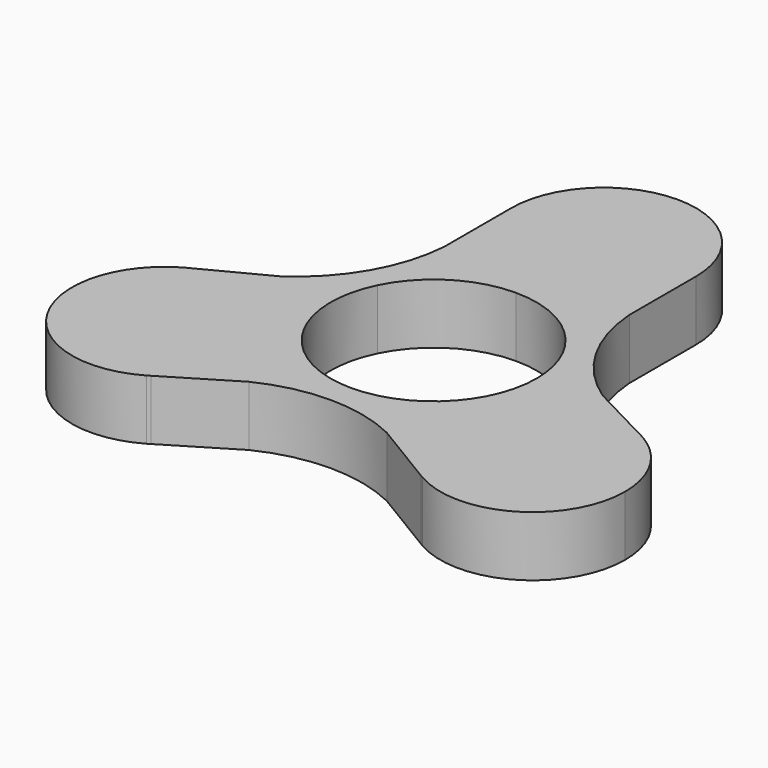
from build123d import *

# Parameters (mm, degrees)
F1_DEPTH = 6.5


# Not quite as in the source:
# - a feature names something its author has since deleted; it is built from what else it names


with BuildPart() as f1:
    # F0 (on Top) → F1 (new body)
    with BuildSketch(Plane.XY):
        with BuildLine():
            Line((10, 13.9658923334), (10, 5.6794919243))
            Line((10, 5.6794919243), (10.6173677664, 4.610179586))
            Line((10.6173677664, 4.610179586), (17.4592921435, 1.0460193523))
            ThreePointArc((17.4592921435, 1.0460193523), (12.2366972109, 6.6440014162), (10, 13.9658923334))
        make_face()
        with BuildLine():
            Line((5, 14.3397459622), (10, 5.6794919243))
            Line((10, 5.6794919243), (10, 13.9658923334))
            Line((10, 13.9658923334), (10, 23))
            ThreePointArc((10, 23), (8.6602540378, 18), (5, 14.3397459622))
        make_face()
        with BuildLine():
            Line((17.4592921435, 1.0460193523), (10.6173677664, 4.610179586))
            Line((10.6173677664, 4.610179586), (14.918584287, -2.8397459622))
            ThreePointArc((14.918584287, -2.8397459622), (19.4852389907, -1.5093938195), (24.1499344795, -2.4393336035))
            Line((24.1499344795, -2.4393336035), (17.4592921435, 1.0460193523))
        make_face()
        with BuildLine():
            Line((-7.4592921435, -15.6551270189), (-0.5795069127, -11.5))
            Line((-0.5795069127, -11.5), (-9.918584287, -11.5))
            ThreePointArc((-9.918584287, -11.5), (-11.1613785992, -16.328182737), (-14.5808539954, -19.9562778652))
            Line((-14.5808539954, -19.9562778652), (-7.4592921435, -15.6551270189))
        make_face()
        with BuildLine():
            Line((0.5795069127, -11.5), (-0.5795069127, -11.5))
            Line((-0.5795069127, -11.5), (-7.4592921435, -15.6551270189))
            ThreePointArc((-7.4592921435, -15.6551270189), (0, -13.9312181655), (7.4592921435, -15.6551270189))
            Line((7.4592921435, -15.6551270189), (0.5795069127, -11.5))
        make_face()
        with BuildLine():
            Line((9.918584287, -11.5), (0.5795069127, -11.5))
            Line((0.5795069127, -11.5), (7.4592921435, -15.6551270189))
            Line((7.4592921435, -15.6551270189), (14.5808539954, -19.9562778652))
            ThreePointArc((14.5808539954, -19.9562778652), (11.1613785992, -16.328182737), (9.918584287, -11.5))
        make_face()
        with BuildLine():
            Line((0, 23), (5, 14.3397459622))
            ThreePointArc((5, 14.3397459622), (8.6602540378, 18), (10, 23))
            Line((10, 23), (0, 23))
        make_face()
        with BuildLine():
            ThreePointArc((24.1499344795, -2.4393336035), (19.4852389907, -1.5093938195), (14.918584287, -2.8397459622))
            Line((14.918584287, -2.8397459622), (19.918584287, -11.5))
            Line((19.918584287, -11.5), (24.918584287, -2.8397459622))
            Line((24.918584287, -2.8397459622), (24.1499344795, -2.4393336035))
        make_face()
        with BuildLine():
            Line((-10, 13.9658923334), (-10, 5.6794919243))
            Line((-10, 5.6794919243), (-5, 14.3397459622))
            ThreePointArc((-5, 14.3397459622), (-8.6602540378, 18), (-10, 23))
            Line((-10, 23), (-10, 13.9658923334))
        make_face()
        with BuildLine():
            Line((-10.6173677664, 4.610179586), (-10, 5.6794919243))
            Line((-10, 5.6794919243), (-10, 13.9658923334))
            ThreePointArc((-10, 13.9658923334), (-12.2366972109, 6.6440014162), (-17.4592921435, 1.0460193523))
            Line((-17.4592921435, 1.0460193523), (-10.6173677664, 4.610179586))
        make_face()
        with BuildLine():
            Line((-14.918584287, -2.8397459622), (-10.6173677664, 4.610179586))
            Line((-10.6173677664, 4.610179586), (-17.4592921435, 1.0460193523))
            Line((-17.4592921435, 1.0460193523), (-24.1499344795, -2.4393336035))
            ThreePointArc((-24.1499344795, -2.4393336035), (-19.4852389907, -1.5093938195), (-14.918584287, -2.8397459622))
        make_face()
        with BuildLine():
            ThreePointArc((-14.5808539954, -19.9562778652), (-11.1613785992, -16.328182737), (-9.918584287, -11.5))
            Line((-9.918584287, -11.5), (-19.918584287, -11.5))
            Line((-19.918584287, -11.5), (-14.918584287, -20.1602540378))
            Line((-14.918584287, -20.1602540378), (-14.5808539954, -19.9562778652))
        make_face()
        with BuildLine():
            Line((19.918584287, -11.5), (9.918584287, -11.5))
            ThreePointArc((9.918584287, -11.5), (11.1613785992, -16.328182737), (14.5808539954, -19.9562778652))
            Line((14.5808539954, -19.9562778652), (14.918584287, -20.1602540378))
            Line((14.918584287, -20.1602540378), (19.918584287, -11.5))
        make_face()
        with BuildLine():
            Line((-5, 14.3397459622), (0, 23))
            Line((0, 23), (-10, 23))
            ThreePointArc((-10, 23), (-8.6602540378, 18), (-5, 14.3397459622))
        make_face()
        with BuildLine():
            Line((-10, 23), (0, 23))
            Line((0, 23), (10, 23))
            ThreePointArc((10, 23), (0, 33), (-10, 23))
        make_face()
        with BuildLine():
            Line((24.918584287, -2.8397459622), (19.918584287, -11.5))
            Line((19.918584287, -11.5), (14.918584287, -20.1602540378))
            ThreePointArc((14.918584287, -20.1602540378), (24.918584287, -20.1602540378), (29.918584287, -11.5))
            ThreePointArc((29.918584287, -11.5), (28.5788383249, -6.5), (24.918584287, -2.8397459622))
        make_face()
        with BuildLine():
            ThreePointArc((24.918584287, -2.8397459622), (24.538599342, -2.6312086003), (24.1499344795, -2.4393336035))
            Line((24.1499344795, -2.4393336035), (24.918584287, -2.8397459622))
        make_face()
        with BuildLine():
            Line((-19.918584287, -11.5), (-14.918584287, -2.8397459622))
            ThreePointArc((-14.918584287, -2.8397459622), (-19.4852389907, -1.5093938195), (-24.1499344795, -2.4393336035))
            Line((-24.1499344795, -2.4393336035), (-24.918584287, -2.8397459622))
            Line((-24.918584287, -2.8397459622), (-19.918584287, -11.5))
        make_face()
        with BuildLine():
            Line((-14.918584287, -20.1602540378), (-19.918584287, -11.5))
            Line((-19.918584287, -11.5), (-24.918584287, -2.8397459622))
            ThreePointArc((-24.918584287, -2.8397459622), (-28.5788383249, -16.5), (-14.918584287, -20.1602540378))
        make_face()
        with BuildLine():
            ThreePointArc((-14.918584287, -20.1602540378), (-14.7487130637, -20.0599317482), (-14.5808539954, -19.9562778652))
            Line((-14.5808539954, -19.9562778652), (-14.918584287, -20.1602540378))
        make_face()
        with BuildLine():
            Line((14.918584287, -20.1602540378), (14.5808539954, -19.9562778652))
            ThreePointArc((14.5808539954, -19.9562778652), (14.7487130637, -20.0599317482), (14.918584287, -20.1602540378))
        make_face()
        with BuildLine():
            Line((-24.918584287, -2.8397459622), (-24.1499344795, -2.4393336035))
            ThreePointArc((-24.1499344795, -2.4393336035), (-24.538599342, -2.6312086003), (-24.918584287, -2.8397459622))
        make_face()
        with BuildLine():
            Line((-0.5795069127, -11.5), (0, -11.15))
            ThreePointArc((0, -11.15), (-9.468682565, -5.8878307111), (-10, 4.9317846668))
            Line((-10, 4.9317846668), (-10.6173677664, 4.610179586))
            Line((-10.6173677664, 4.610179586), (-14.918584287, -2.8397459622))
            ThreePointArc((-14.918584287, -2.8397459622), (-11.2583302492, -6.5), (-9.918584287, -11.5))
            Line((-9.918584287, -11.5), (-0.5795069127, -11.5))
        make_face()
        with BuildLine():
            Line((-19.918584287, -11.5), (-9.918584287, -11.5))
            ThreePointArc((-9.918584287, -11.5), (-11.2583302492, -6.5), (-14.918584287, -2.8397459622))
            Line((-14.918584287, -2.8397459622), (-19.918584287, -11.5))
        make_face()
        Polygon((-10.6173677664, 4.610179586), (-10, 4.9317846668), (-10, 5.6794919243), align=None)
        with BuildLine():
            ThreePointArc((-10, 4.9317846668), (-5.8878307111, 9.468682565), (0, 11.15))
            Line((0, 11.15), (0, 13))
            ThreePointArc((0, 13), (-2.588190451, 13.3407417371), (-5, 14.3397459622))
            Line((-5, 14.3397459622), (-10, 5.6794919243))
            Line((-10, 5.6794919243), (-10, 4.9317846668))
        make_face()
        with BuildLine():
            ThreePointArc((-5, 14.3397459622), (-2.588190451, 13.3407417371), (0, 13))
            Line((0, 13), (0, 23))
            Line((0, 23), (-5, 14.3397459622))
        make_face()
        with BuildLine():
            Line((0, 23), (0, 13))
            ThreePointArc((0, 13), (2.588190451, 13.3407417371), (5, 14.3397459622))
            Line((5, 14.3397459622), (0, 23))
        make_face()
        with BuildLine():
            ThreePointArc((0, 11.15), (5.8878307111, 9.468682565), (10, 4.9317846668))
            Line((10, 4.9317846668), (10, 5.6794919243))
            Line((10, 5.6794919243), (5, 14.3397459622))
            ThreePointArc((5, 14.3397459622), (2.588190451, 13.3407417371), (0, 13))
            Line((0, 13), (0, 11.15))
        make_face()
        Polygon((10, 5.6794919243), (10, 4.9317846668), (10.6173677664, 4.610179586), align=None)
        with BuildLine():
            ThreePointArc((10, 4.9317846668), (10.8586946729, 2.5320446284), (11.15, 0))
            ThreePointArc((11.15, 0), (7.8842406102, -7.8842406102), (0, -11.15))
            Line((0, -11.15), (0.5795069127, -11.5))
            Line((0.5795069127, -11.5), (9.918584287, -11.5))
            ThreePointArc((9.918584287, -11.5), (11.2583302492, -6.5), (14.918584287, -2.8397459622))
            Line((14.918584287, -2.8397459622), (10.6173677664, 4.610179586))
            Line((10.6173677664, 4.610179586), (10, 4.9317846668))
        make_face()
        with BuildLine():
            Line((19.918584287, -11.5), (14.918584287, -2.8397459622))
            ThreePointArc((14.918584287, -2.8397459622), (11.2583302492, -6.5), (9.918584287, -11.5))
            Line((9.918584287, -11.5), (19.918584287, -11.5))
        make_face()
        Polygon((0.5795069127, -11.5), (0, -11.15), (-0.5795069127, -11.5), align=None)
    extrude(amount=F1_DEPTH)


solid = f1.part
